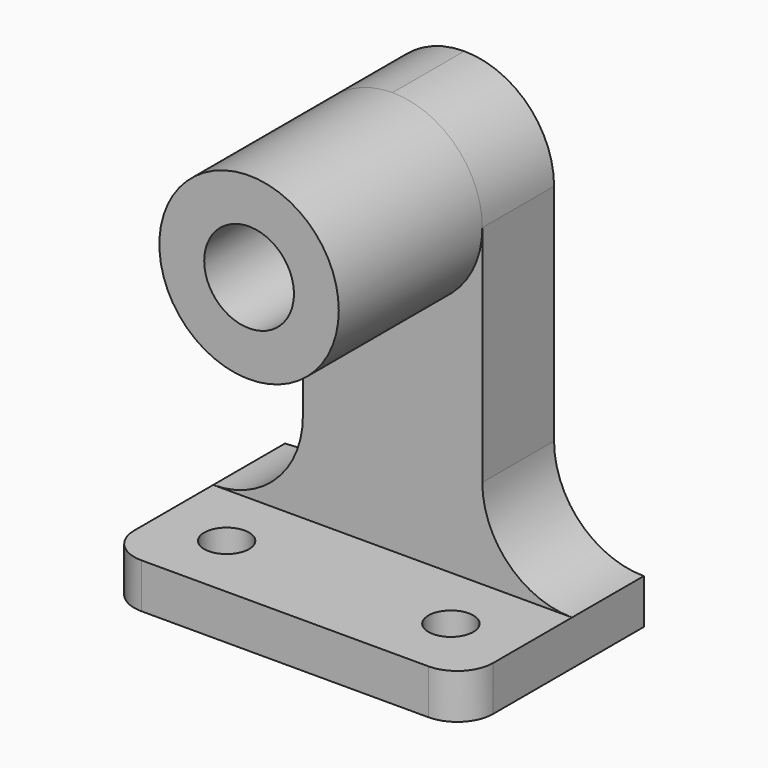
from build123d import *

# Parameters (mm, degrees)
F0_W     = 50.8
F0_H     = 52.8410717415
F0_H_2   = 10.6589282585
F1_DEPTH = 12.7
F2_W     = 50.8
F2_H     = 6.35
F3_DEPTH = 19.05
F5_DEPTH = 25.4
F7_DEPTH = 25.4
F9_D     = 12.7
F10_R    = 5.08
F12_D    = 6.35


with BuildPart() as f1:
    # F0 (on Front) → F1 (new body)
    with BuildSketch(Plane.XZ):
        with Locations((-40.9050544952, 43.3130595229)):
            Rectangle(F0_W, F0_H)
        with Locations((-40.9050544952, 11.5630595229)):
            Rectangle(F0_W, F0_H_2)
    extrude(amount=F1_DEPTH)

    # F2 (on face) → F3 (join)
    with BuildSketch(Plane.XZ.offset(12.7)):
        with Locations((-40.9050544952, 9.4085953936)):
            Rectangle(F2_W, F2_H)
    extrude(amount=F3_DEPTH)

    # F4 (on face) → F5 (cut)
    with BuildSketch(Plane.XZ.offset(12.7)):
        with BuildLine():
            Line((-53.6050544952, 25.2835953936), (-53.6050544952, 57.0335953936))
            ThreePointArc((-53.6050544952, 57.0335953936), (-49.8853106163, 66.0138515147), (-40.9050544952, 69.7335953936))
            Line((-40.9050544952, 69.7335953936), (-66.3050544952, 69.7335953936))
            Line((-66.3050544952, 69.7335953936), (-66.3050544952, 12.5835953936))
            ThreePointArc((-66.3050544952, 12.5835953936), (-57.3247983741, 16.3033392725), (-53.6050544952, 25.2835953936))
        make_face()
        with BuildLine():
            ThreePointArc((-40.9050544952, 69.7335953936), (-31.9247983741, 66.0138515147), (-28.2050544952, 57.0335953936))
            Line((-28.2050544952, 57.0335953936), (-28.2050544952, 25.2835953936))
            ThreePointArc((-28.2050544952, 25.2835953936), (-24.4853106163, 16.3033392725), (-15.5050544952, 12.5835953936))
            Line((-15.5050544952, 12.5835953936), (-15.5050544952, 69.7335953936))
            Line((-15.5050544952, 69.7335953936), (-40.9050544952, 69.7335953936))
        make_face()
    extrude(amount=-F5_DEPTH, mode=Mode.SUBTRACT)

    # F6 (on face) → F7 (join)
    with BuildSketch(Plane.XZ.offset(12.7)):
        with BuildLine():
            ThreePointArc((-53.6050544952, 57.0335953936), (-40.9050544952, 44.3335953936), (-28.2050544952, 57.0335953936))
            ThreePointArc((-28.2050544952, 57.0335953936), (-40.9050544952, 69.7335953936), (-53.6050544952, 57.0335953936))
        make_face()
    extrude(amount=F7_DEPTH)

    # F9 (through all)
    with Locations(Plane.XZ.offset(38.1)):
        with Locations((-40.9050544952, 57.0335953936)):
            Hole(F9_D / 2)

    # F10
    f10_edges = [f1.edges().sort_by_distance(p)[0] for p in [
        (-66.305054, -31.75, 9.408595),
        (-15.505054, -31.75, 9.408595),
    ]]
    fillet(f10_edges, radius=F10_R)

    # F12 (through all)
    with Locations(Plane.XY.offset(12.5835953936)):
        with Locations((-56.7800544952, -22.225), (-25.0300544952, -22.225)):
            Hole(F12_D / 2)


solid = f1.part
